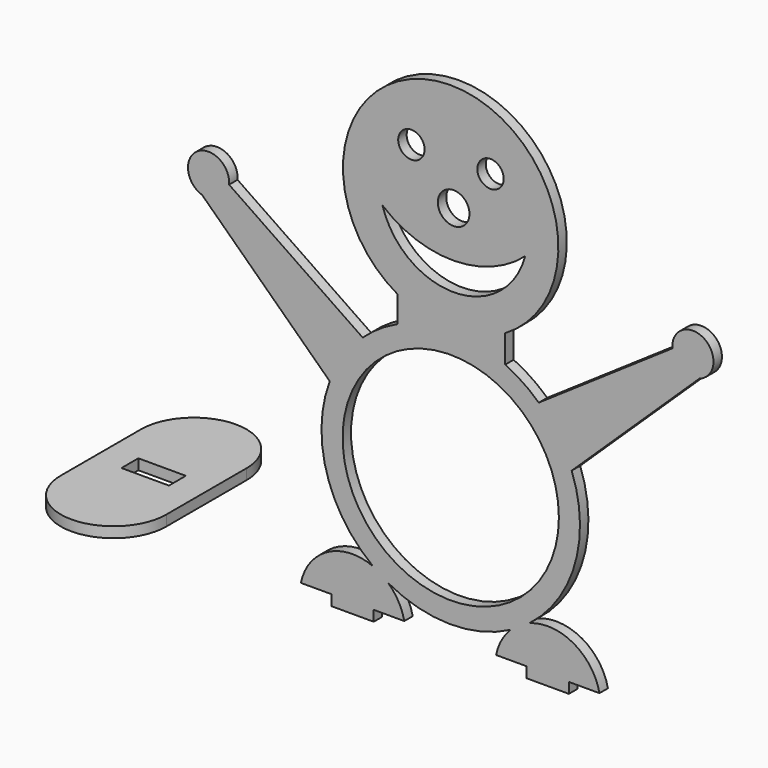
from build123d import *

# Parameters (mm, degrees)
F0_R     = 20.5
F0_R_2   = 2.5
F0_R_3   = 3
F0_W     = 8
F0_H     = 2
F1_DEPTH = 2
F2_W     = 9
F2_H     = 4
F3_DEPTH = 2


# Not quite as in the source:
# - a feature names something its author has since deleted; it is built from what else it names


with BuildPart() as f1:
    # F0 (on Front) → F1 (new body)
    with BuildSketch(Plane.XZ):
        with BuildLine():
            Line((-10.0518541032, 27.3076325654), (-10.0518541032, 22.3430129814))
            ThreePointArc((-10.0518541032, 22.3430129814), (-10.1932123132, 22.2788783995), (-10.3341613447, 22.2138494931))
            ThreePointArc((-10.3341613447, 22.2138494931), (-13.6806146729, 20.3246348595), (-16.6904854096, 17.9353755688))
            Line((-16.6904854096, 17.9353755688), (-42.0114619192, 35.2237376845))
            ThreePointArc((-42.0114619192, 35.2237376845), (-48.0533290823, 38.8096157049), (-47.1334807155, 31.8442328026))
            Line((-47.1334807155, 31.8442328026), (-22.9334270643, 8.620204353))
            ThreePointArc((-22.9334270643, 8.620204353), (-22.9337135716, 8.6194420827), (-22.9340000535, 8.6186798029))
            ThreePointArc((-22.9340000535, 8.6186798029), (-22.9521939831, 8.5701103472), (-22.9702850527, 8.5215024848))
            ThreePointArc((-22.9702850527, 8.5215024848), (-23.543020169, -6.7805752945), (-14.9189118524, -19.4338897069))
            ThreePointArc((-14.9189118524, -19.4338897069), (-14.8050096032, -19.5208014858), (-14.6906010516, -19.6070456914))
            ThreePointArc((-14.6906010516, -19.6070456914), (-23.2540973357, -19.9569387989), (-28.4014469494, -26.809725513))
            Line((-28.4014469494, -26.809725513), (-22.6034879783, -26.809725513))
            Line((-22.6034879783, -26.809725513), (-14.6034879783, -26.809725513))
            Line((-14.6034879783, -26.809725513), (-8.8055290071, -26.809725513))
            ThreePointArc((-8.8055290071, -26.809725513), (-9.8942672501, -23.8955140495), (-11.8258820824, -21.4568989598))
            ThreePointArc((-11.8258820824, -21.4568989598), (-0.2678936029, -24.4985353239), (11.3538442484, -21.7103712724))
            ThreePointArc((11.3538442484, -21.7103712724), (9.5986412165, -24.0560459597), (8.5985530506, -26.809725513))
            Line((8.5985530506, -26.809725513), (14.3965120217, -26.809725513))
            Line((14.3965120217, -26.809725513), (22.3965120217, -26.809725513))
            Line((22.3965120217, -26.809725513), (28.1944709929, -26.809725513))
            ThreePointArc((28.1944709929, -26.809725513), (23.2532055786, -20.0682995598), (14.9189118524, -19.4338897069))
            ThreePointArc((14.9189118524, -19.4338897069), (23.5575452615, -6.7299376857), (22.9334270643, 8.620204353))
            Line((22.9334270643, 8.620204353), (47.1334807155, 31.8442328026))
            ThreePointArc((47.1334807155, 31.8442328026), (48.0533290823, 38.8096157049), (42.0114619192, 35.2237376845))
            Line((42.0114619192, 35.2237376845), (16.6904854096, 17.9353755688))
            ThreePointArc((16.6904854096, 17.9353755688), (13.6806146729, 20.3246348595), (10.3341613447, 22.2138494931))
            Line((10.3341613447, 22.2138494931), (10.3341613447, 27.4808270977))
            ThreePointArc((10.3341613447, 27.4808270977), (-0.1825659758, 65.4979309649), (-10.0518541032, 27.3076325654))
        make_face()
        Circle(F0_R, mode=Mode.SUBTRACT)
        with Locations((-7.4579087086, 53.1332939863)):
            Circle(F0_R_2, mode=Mode.SUBTRACT)
        with BuildLine():
            ThreePointArc((14.1213098541, 41.5384881198), (0.7163199464, 31.1055576115), (-12.9332384095, 41.2164106965))
            ThreePointArc((-12.9332384095, 41.2164106965), (0.6534592539, 36.3858645098), (14.1213098541, 41.5384881198))
        make_face(mode=Mode.SUBTRACT)
        with Locations((0.5491401715, 45.1486819078)):
            Circle(F0_R_3, mode=Mode.SUBTRACT)
        with Locations((7.5420912914, 53.1332939863)):
            Circle(F0_R_2, mode=Mode.SUBTRACT)
        with Locations((18.3965120217, -27.809725513)):
            Rectangle(F0_W, F0_H)
        with Locations((-18.6034879783, -27.809725513)):
            Rectangle(F0_W, F0_H)
    extrude(amount=F1_DEPTH)


with BuildPart() as f3:
    # F2 (on Top) → F3 (new body)
    with BuildSketch(Plane.XY):
        with BuildLine():
            ThreePointArc((-23.0774022639, -21.5484288931), (-33.0774022639, -11.5484288931), (-43.0774022639, -21.5484288931))
            Line((-43.0774022639, -21.5484288931), (-43.0774022639, -40.5484288931))
            ThreePointArc((-43.0774022639, -40.5484288931), (-33.0774022639, -50.5484288931), (-23.0774022639, -40.5484288931))
            Line((-23.0774022639, -40.5484288931), (-23.0774022639, -21.5484288931))
        make_face()
        with Locations((-33.0774022639, -31.0484288931)):
            Rectangle(F2_W, F2_H, mode=Mode.SUBTRACT)
    extrude(amount=F3_DEPTH)


solid = Compound([f1.part, f3.part])
